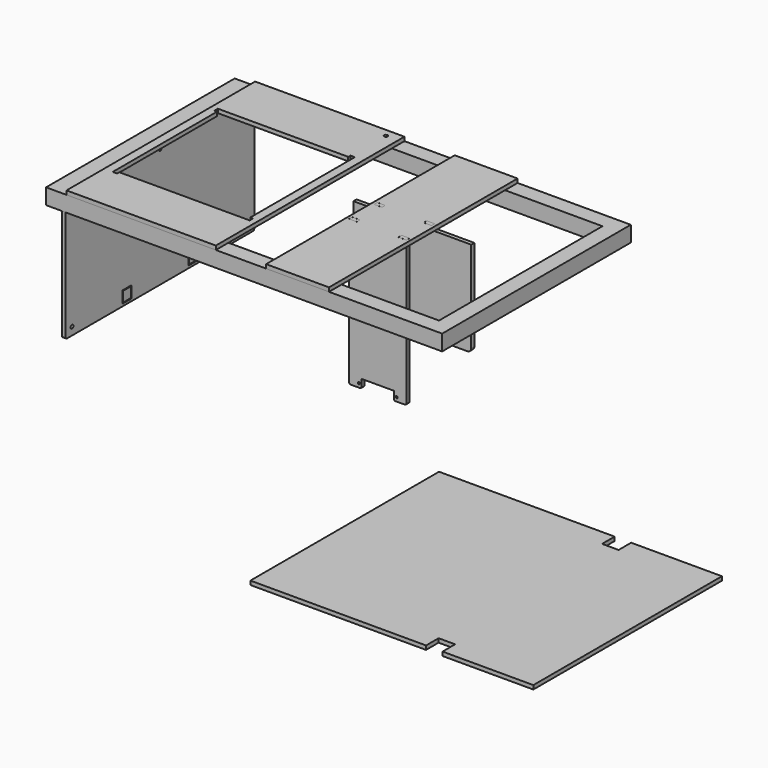
from build123d import *

# Parameters (mm, degrees)
F2_R      = 1.4
F3_DEPTH  = 5
F0_R      = 1.4
F4_DEPTH  = 5
F9_W      = 464
F9_H      = 20
F9_W_2    = 20
F9_H_2    = 260
F10_DEPTH = 20
F11_DEPTH = 5
F16_W     = 190
F16_H     = 260
F16_H_2   = 20
F16_R     = 2.25
F17_DEPTH = 5
F18_W     = 80
F18_H     = 300
F18_W_2   = 10.1
F18_H_2   = 5.1
F19_DEPTH = 5
F15_R     = 2.25
F15_W     = 15
F15_H     = 15
F22_DEPTH = 5
F21_W     = 13
F21_H     = 13
F23_DEPTH = 10
F24_W     = 122
F24_H     = 17
F24_W_2   = 5
F24_H_2   = 10
F25_DEPTH = 5
F27_R     = 0.9
F28_DEPTH = 5
F30_R     = 1.4
F31_DEPTH = 5
F32_R     = 4.95
F33_DEPTH = 5


# Not quite as in the source:
# - a feature of the source that left no trace in its solid (it failed there, or was rolled back) is left out
# - a feature names something its author has since deleted; it is built from what else it names


with BuildPart() as f3:
    # F2 (on offset) → F3 (new body)
    with BuildSketch(Plane.XZ.offset(35)):
        with BuildLine():
            ThreePointArc((-26.5, 2), (-25.9142135624, 0.5857864376), (-24.5, 0))
            Line((-24.5, 0), (-12.5, 0))
            ThreePointArc((-12.5, 0), (-11.0857864376, 0.5857864376), (-10.5, 2))
            Line((-10.5, 2), (-10.5, 11))
            Line((-10.5, 11), (30.5, 11))
            Line((30.5, 11), (30.5, 2))
            ThreePointArc((30.5, 2), (31.0857864376, 0.5857864376), (32.5, 0))
            Line((32.5, 0), (44.5, 0))
            ThreePointArc((44.5, 0), (45.9142135624, 0.5857864376), (46.5, 2))
            Line((46.5, 2), (46.5, 100))
            Line((46.5, 100), (46.5, 185))
            Line((46.5, 185), (36.5, 185))
            Line((36.5, 185), (36.5, 180))
            Line((36.5, 180), (-16.5, 180))
            Line((-16.5, 180), (-16.5, 185))
            Line((-16.5, 185), (-26.5, 185))
            Line((-26.5, 185), (-26.5, 180))
            Line((-26.5, 180), (-26.5, 2))
        make_face()
        with Locations((-14, 5)):
            Circle(F2_R, mode=Mode.SUBTRACT)
        with Locations((34, 5)):
            Circle(F2_R, mode=Mode.SUBTRACT)
    extrude(amount=F3_DEPTH)


with BuildPart() as f4:
    # F0 (on Front) → F4 (new body)
    with BuildSketch(Plane.XZ):
        with BuildLine():
            Line((-53, 180), (-53, 64))
            ThreePointArc((-53, 64), (-51.5355339059, 60.4644660941), (-48, 59))
            Line((-48, 59), (92, 59))
            ThreePointArc((92, 59), (95.5355339059, 60.4644660941), (97, 64))
            Line((97, 64), (97, 180))
            Line((97, 180), (46.5, 180))
            Line((46.5, 180), (46.5, 185))
            Line((46.5, 185), (36.5, 185))
            Line((36.5, 185), (36.5, 180))
            Line((36.5, 180), (-16.5, 180))
            Line((-16.5, 180), (-16.5, 185))
            Line((-16.5, 185), (-26.5, 185))
            Line((-26.5, 185), (-26.5, 180))
            Line((-26.5, 180), (-53, 180))
        make_face()
        with Locations((-45, 67)):
            Circle(F0_R, mode=Mode.SUBTRACT)
        with Locations((89, 78)):
            Circle(F0_R, mode=Mode.SUBTRACT)
    extrude(amount=-F4_DEPTH)


with BuildPart() as f10:
    # F9 (on offset) → F10 (new body)
    with BuildSketch(Plane.XY.offset(160)):
        with Locations((-58, 122.5)):
            Rectangle(F9_W, F9_H)
        with Locations((-300, -17.5)):
            Rectangle(F9_W_2, F9_H_2)
        with Locations((-300, 122.5)):
            Rectangle(F9_W_2, F9_H)
        with Locations((184, -17.5)):
            Rectangle(F9_W_2, F9_H_2)
        with Locations((184, 122.5)):
            Rectangle(F9_W_2, F9_H)
        with Locations((-300, -157.5)):
            Rectangle(F9_W_2, F9_H)
        with Locations((-58, -157.5)):
            Rectangle(F9_W, F9_H)
        with Locations((184, -157.5)):
            Rectangle(F9_W_2, F9_H)
    extrude(amount=F10_DEPTH)


with BuildPart() as f11:
    # F7 (on offset) → F11 (new body)
    with BuildSketch(Plane.XY.offset(-176)):
        Polygon((173.5, 112.5), (173.5, 132.5), (-50, 132.5), (-50, -167.5), (173.5, -167.5), (173.5, -147.5), (194.5, -147.5), (194.5, -167.5), (310, -167.5), (310, 132.5), (194.5, 132.5), (194.5, 112.5), align=None)
    extrude(amount=-F11_DEPTH)


with BuildPart() as f17:
    # F16 (on face) → F17 (new body)
    with BuildSketch(Plane.XY.offset(180)):
        with Locations((-189, -17.5)):
            Rectangle(F16_W, F16_H)
        Polygon((-273, -107.75), (-273, -104.25), (-273, 58.25), (-276.5, 58.25), (-276.5, 63.75), (-273, 63.75), (-110.5, 63.75), (-110.5, 67.25), (-105, 67.25), (-105, 63.75), (-105, -98.75), (-101.5, -98.75), (-101.5, -104.25), (-105, -104.25), (-267.5, -104.25), (-267.5, -107.75), align=None, mode=Mode.SUBTRACT)
        with Locations((-189, -157.5)):
            Rectangle(F16_W, F16_H_2)
        with Locations((-189, 122.5)):
            Rectangle(F16_W, F16_H_2)
        with Locations((-109.6, 122.5)):
            Circle(F16_R, mode=Mode.SUBTRACT)
    extrude(amount=F17_DEPTH)


with BuildPart() as f19:
    # F18 (on face) → F19 (new body)
    with BuildSketch(Plane.XY.offset(180)):
        with Locations((10, -17.5)):
            Rectangle(F18_W, F18_H)
        with Locations((-21.5, -37.5)):
            Rectangle(F18_W_2, F18_H_2, mode=Mode.SUBTRACT)
        with Locations((41.5, -37.5)):
            Rectangle(F18_W_2, F18_H_2, mode=Mode.SUBTRACT)
        with Locations((-21.5, 2.5)):
            Rectangle(F18_W_2, F18_H_2, mode=Mode.SUBTRACT)
        with Locations((41.5, 2.5)):
            Rectangle(F18_W_2, F18_H_2, mode=Mode.SUBTRACT)
    extrude(amount=F19_DEPTH)


with BuildPart() as f22:
    # F15 (on face) → F22 (new body)
    with BuildSketch(Plane.YZ.offset(-290)):
        with BuildLine():
            ThreePointArc((-167.5, 20), (-166.9142135624, 18.5857864376), (-165.5, 18))
            Line((-165.5, 18), (130.5, 18))
            ThreePointArc((130.5, 18), (131.9142135624, 18.5857864376), (132.5, 20))
            Line((132.5, 20), (132.5, 160))
            Line((132.5, 160), (112, 160))
            Line((112, 160), (112, 180))
            Line((112, 180), (-147, 180))
            Line((-147, 180), (-147, 160))
            Line((-147, 160), (-167.5, 160))
            Line((-167.5, 160), (-167.5, 20))
        make_face()
        with Locations((-157.5, 28)):
            Circle(F15_R, mode=Mode.SUBTRACT)
        with Locations((-70, 28.5)):
            Rectangle(F15_W, F15_H, mode=Mode.SUBTRACT)
        with Locations((35, 28.5)):
            Rectangle(F15_W, F15_H, mode=Mode.SUBTRACT)
        with Locations((122.5, 28)):
            Circle(F15_R, mode=Mode.SUBTRACT)
        with Locations((-17.5, 170)):
            Circle(F15_R, mode=Mode.SUBTRACT)
    extrude(amount=F22_DEPTH)

    # F27 (on offset) → F28 (join)
    with BuildSketch(Plane.XZ.offset(15)):
        Polygon((-315, 40), (-290, 40), (-285, 40), (-285, 45), (-290, 45), (-290, 55), (-285, 55), (-285, 60), (-290, 60), (-315, 60), align=None)
        with Locations((-310, 48.5)):
            Circle(F27_R, mode=Mode.SUBTRACT)
    extrude(amount=-F28_DEPTH)

    # F30 (on offset) → F31 (join)
    with BuildSketch(Plane.XZ.offset(-5)):
        with BuildLine():
            ThreePointArc((-308, 115.9), (-309.4142135624, 115.3142135624), (-310, 113.9))
            Line((-310, 113.9), (-310, 101.9))
            ThreePointArc((-310, 101.9), (-309.4142135624, 100.4857864376), (-308, 99.9))
            Line((-308, 99.9), (-299, 99.9))
            Line((-299, 99.9), (-299, 58.9))
            Line((-299, 58.9), (-308, 58.9))
            ThreePointArc((-308, 58.9), (-309.4142135624, 58.3142135624), (-310, 56.9))
            Line((-310, 56.9), (-310, 44.9))
            ThreePointArc((-310, 44.9), (-309.4142135624, 43.4857864376), (-308, 42.9))
            Line((-308, 42.9), (-290, 42.9))
            Line((-290, 42.9), (-290, 115.9))
            Line((-290, 115.9), (-308, 115.9))
        make_face()
        with Locations((-305, 55.4)):
            Circle(F30_R, mode=Mode.SUBTRACT)
        with Locations((-305, 103.4)):
            Circle(F30_R, mode=Mode.SUBTRACT)
    extrude(amount=-F31_DEPTH)


with BuildPart() as f23:
    # F21 (on offset) → F23 (new body)
    with BuildSketch(Plane.YZ.offset(-295)):
        with Locations((35, 28.5)):
            Rectangle(F21_W, F21_H)
    extrude(amount=F23_DEPTH)


with BuildPart() as f23b:
    # F21 (on offset) → F23, piece 2 (new body)
    with BuildSketch(Plane.YZ.offset(-295)):
        with Locations((-70, 28.5)):
            Rectangle(F21_W, F21_H)
    extrude(amount=F23_DEPTH)


with BuildPart() as f25:
    # F24 (on offset) → F25 (new body)
    with BuildSketch(Plane.YZ.offset(-295)):
        with Locations((-17.5, 28.5)):
            Rectangle(F24_W, F24_H)
        with Locations((-17.5, 28.5)):
            Rectangle(F24_W_2, F24_H_2, mode=Mode.SUBTRACT)
    extrude(amount=-F25_DEPTH)


with BuildPart() as f33:
    # F32 (on offset) → F33 (new body)
    with BuildSketch(Plane.XZ.offset(15)):
        Polygon((-318, 23.5), (-295, 23.5), (-295, 33.5), (-302, 33.5), (-302, 98.5), (-318, 98.5), align=None)
        with Locations((-310, 48.5)):
            Circle(F32_R, mode=Mode.SUBTRACT)
        with Locations((-310, 88.5)):
            Circle(F32_R, mode=Mode.SUBTRACT)
    extrude(amount=F33_DEPTH)


solid = Compound([f3.part, f4.part, f10.part, f11.part, f17.part, f19.part, f22.part, f23.part, f23b.part, f25.part, f33.part])
